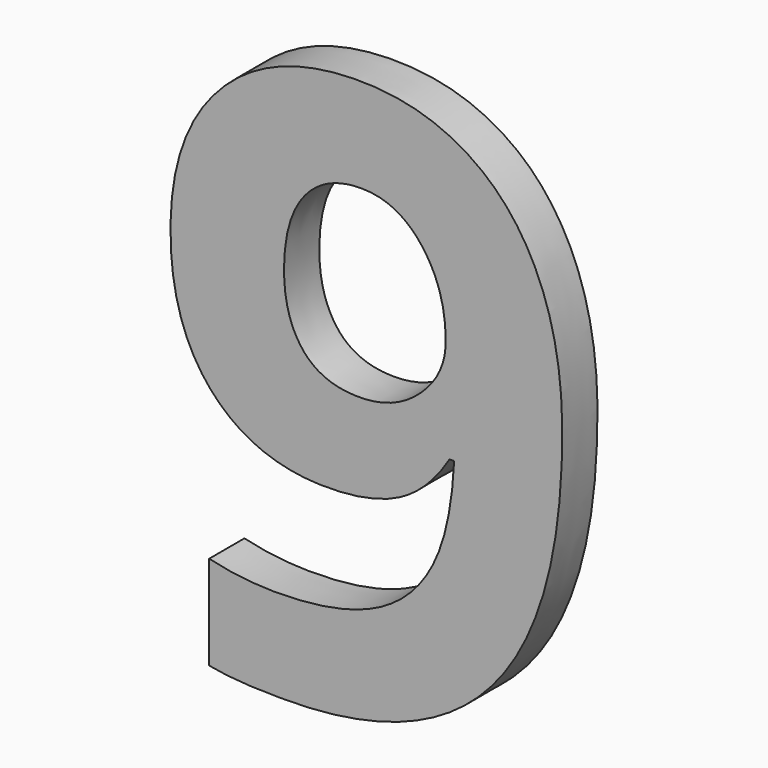
from build123d import *

# Parameters (mm, degrees)
F0_TEXT_SIZE = 70.5555555556
F1_DEPTH     = 4


# Not quite as in the source:
# - Text() gives the source's letters only with a copy of the font that has no kerning and outlines rounded to 1/6400 em; it was checked with that copy


with BuildPart() as f1:
    # F0 (on Front) → F1 (new body)
    with BuildSketch(Plane.XZ):
        with Locations((0, 0)):
            Text('9', F0_TEXT_SIZE, font='Open Sans', font_style=FontStyle.BOLD, text_align=(TextAlign.LEFT, TextAlign.BOTTOM))
    extrude(amount=F1_DEPTH)


solid = f1.part
